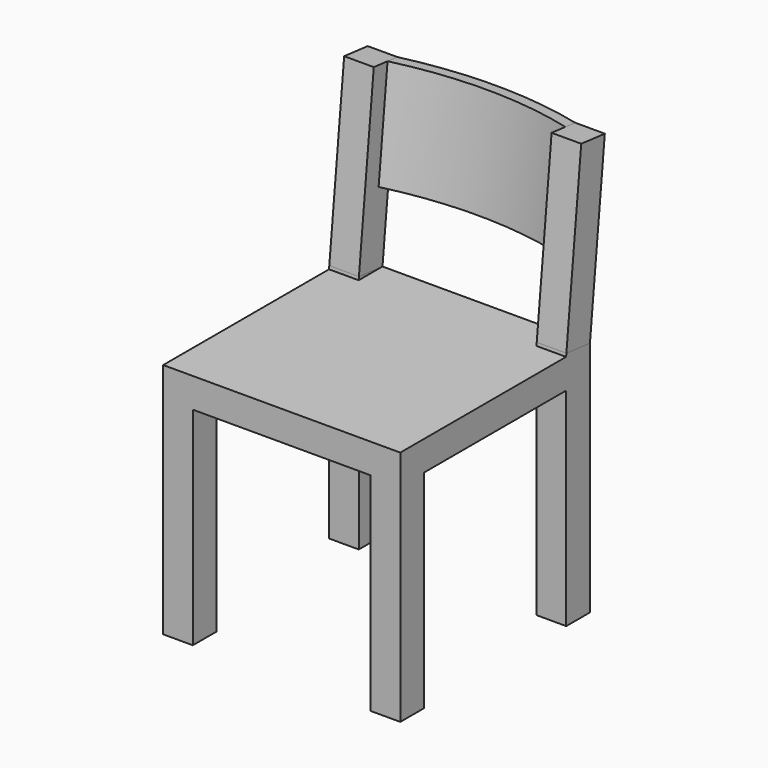
from build123d import *

# Parameters (mm, degrees)
F0_W      = 10160
F0_H      = 10160
F1_DEPTH  = 10160
F2_W      = 7620
F2_H      = 8890
F3_DEPTH  = 12979.4
F4_W      = 7620
F4_H      = 8890
F5_DEPTH  = 15138.4
F10_W     = 10160
F10_H     = 7620
F11_DEPTH = 1270
F12_W     = 7620
F12_H     = 7620
F13_DEPTH = 5130.8
F15_W     = 1270
F15_H     = 1270
F16_DEPTH = 170.18
F14_W     = 1270
F14_H     = 1270
F17_DEPTH = 208.28
F19_DEPTH = 4572


with BuildPart() as f1:
    # F0 (on Top) → F1 (new body)
    with BuildSketch(Plane.XY):
        Rectangle(F0_W, F0_H)
    extrude(amount=F1_DEPTH)

    # F2 (on face) → F3 (cut)
    with BuildSketch(Plane.XZ.offset(5080)):
        with Locations((0, 4445)):
            Rectangle(F2_W, F2_H)
    extrude(amount=-F3_DEPTH, mode=Mode.SUBTRACT)

    # F4 (on face) → F5 (cut)
    with BuildSketch(Plane(origin=(-5080, 0, 0), x_dir=(0, -1, 0), z_dir=(-1, 0, 0))):
        with Locations((0, 4445)):
            Rectangle(F4_W, F4_H)
    extrude(amount=-F5_DEPTH, mode=Mode.SUBTRACT)

    # F15 (on face) → F16 (join)
    with BuildSketch(Plane(origin=(0, 1111.6964834904, 10577.0855064048), x_dir=(1, 0, 0), z_dir=(0, -0.1045284633, -0.9945218954))):
        with Locations((4445, -3355.1620416715)):
            Rectangle(F15_W, F15_H)
    extrude(amount=F16_DEPTH)

    # F14 (on face) → F17 (join)
    with BuildSketch(Plane(origin=(0, 1111.6964834904, 10577.0855064048), x_dir=(1, 0, 0), z_dir=(0, -0.1045284633, -0.9945218954))):
        with Locations((-4445, -3355.1620416715)):
            Rectangle(F14_W, F14_H)
    extrude(amount=F17_DEPTH)


with BuildPart() as f11:
    # F10 (on face) → F11 (new body)
    with BuildSketch(Plane(origin=(0, 3968.3035165096, -417.0855064048), x_dir=(-1, 0, 0), z_dir=(0, 0.9945218954, -0.1045284633))):
        with Locations((0, 14445.3470503413)):
            Rectangle(F10_W, F10_H)
    extrude(amount=-F11_DEPTH)

    # F12 (on face) → F13 (cut)
    with BuildSketch(Plane(origin=(0, 2705.2607093919, -284.3343580549), x_dir=(1, 0, 0), z_dir=(0, -0.9945218954, 0.1045284633))):
        with Locations((0, 14445.3470503413)):
            Rectangle(F12_W, F12_H)
    extrude(amount=-F13_DEPTH, mode=Mode.SUBTRACT)


with BuildPart() as f19:
    # F18 (on face) → F19 (new body)
    with BuildSketch(Plane(origin=(0, 1908.2033735899, 18155.3423491111), x_dir=(1, 0, 0), z_dir=(0, 0.1045284633, 0.9945218954))):
        with BuildLine():
            Line((3810, 3460.9414873997), (3810, 3990.1620416715))
            ThreePointArc((3810, 3990.1620416715), (0, 4524.6190016034), (-3810, 3990.1620416715))
            Line((-3810, 3990.1620416715), (-3810, 3460.9414873997))
            ThreePointArc((-3810, 3460.9414873997), (0, 4016.6190016034), (3810, 3460.9414873997))
        make_face()
    extrude(amount=-F19_DEPTH)


solid = Compound([f1.part, f11.part, f19.part])
